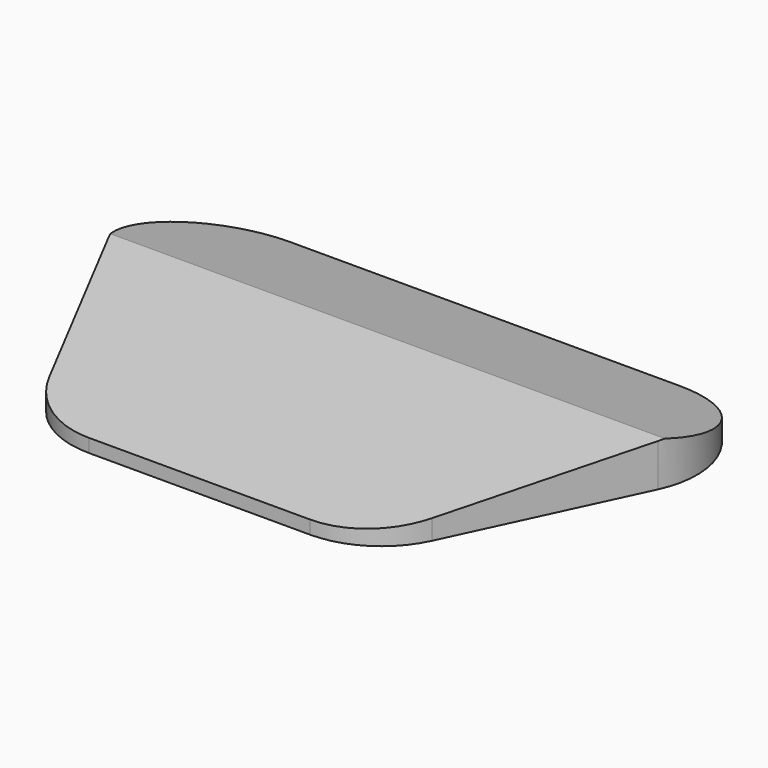
from build123d import *

# Parameters (mm, degrees)
F1_DEPTH    = 5.08
F2_SIZE2    = 3.556
F2_SIZE     = 14.478
F3_T1_DEPTH = 183.3449978003
F4_R        = 10.16


# Not quite as in the source:
# - a fillet or chamfer that OpenCascade refuses, or shapes differently, is made with other operations: its cross-section is extruded or revolved along the edge and cut away or added


with BuildPart() as f1:
    # F0 (on Top) → F1 (new body)
    with BuildSketch(Plane.XY):
        Polygon((-38.1, 23.2852384394), (-19.05, -17.3547615606), (19.05, -17.3547615606), (38.1, 23.2852384394), align=None)
    extrude(amount=F1_DEPTH)

    # F2
    f2_edges = [f1.edges().sort_by_distance(p)[0] for p in [
        (0, 23.285238, 5.08),
    ]]
    f2_side = f1.faces().sort_by_distance((0, 5.223016, 5.08))[0]
    chamfer(f2_edges, length=F2_SIZE, length2=F2_SIZE2, reference=f2_side)

    # F3: chamfer of 27.94 x 3.556 on 1 edges, made by hand

    # F3_s2 → F3_t1 (cut)
    with BuildSketch(Plane.YZ.offset(-91.6724989001)):
        Polygon((10.5852384394, 5.08), (-17.3547615606, 1.524), (-17.3547615606, 5.08), align=None)
    extrude(amount=F3_T1_DEPTH, mode=Mode.SUBTRACT)

    # F4
    f4_edges = [f1.edges().sort_by_distance(p)[0] for p in [
        (19.05, -17.354762, 0.762),
        (-19.05, -17.354762, 0.762),
        (38.1, 23.285238, 0.762),
        (-38.1, 23.285238, 0.762),
    ]]
    fillet(f4_edges, radius=F4_R)


solid = f1.part
